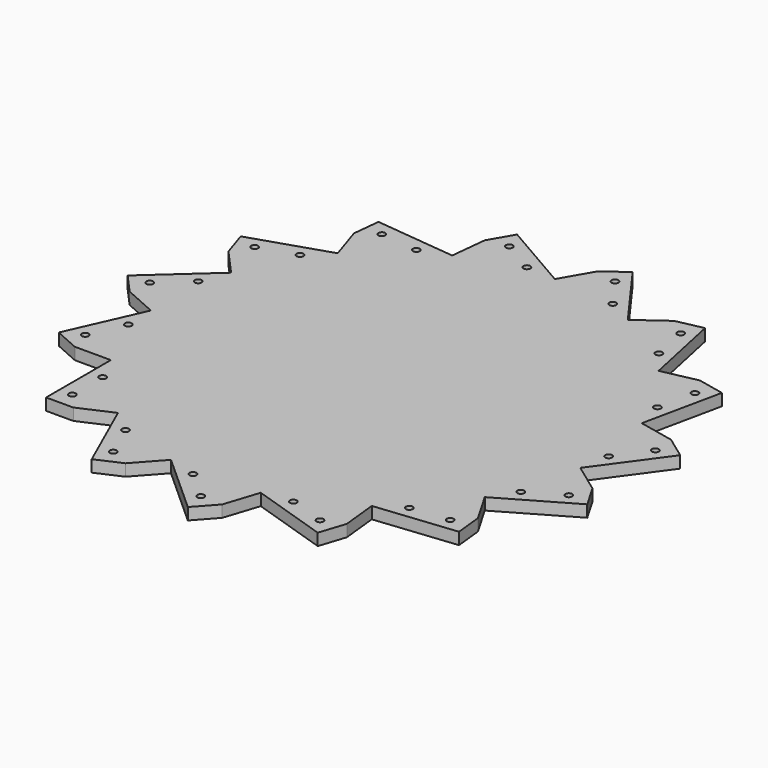
from build123d import *

# Parameters (mm, degrees)
F0_R     = 1.45
F1_DEPTH = 5


# Not quite as in the source:
# - ends of sketch curves that miss each other by under 0.0002 mm in the source are joined


with BuildPart() as f1:
    # F0 (on Top) → F1 (new body)
    with BuildSketch(Plane.XY):
        Polygon((-0.3545266845, 90.9670817697), (-29.9807621135, 108.0717967697), (-35.7307621135, 98.1125046262), (-37.3235262825, 82.9583658326), (-71.3455488748, 86.5342244993), (-72.5476262023, 75.0972227026), (-67.8389451324, 60.6053924919), (-100.3740420816, 50.0340986743), (-96.8203466463, 39.0969487369), (-86.6243940714, 27.7731962067), (-112.046951543, 4.8826226429), (-104.3519495698, -3.6635428501), (-90.4316983176, -9.8612380143), (-104.345925168, -41.1131032006), (-93.8401524051, -45.790574596), (-78.6025403784, -45.790574596), (-78.6025403784, -80), (-67.1025403784, -80), (-53.1822891262, -73.8023048358), (-39.2680622758, -105.0541700222), (-28.7622895129, -100.3766986268), (-18.5663369381, -89.0529460966), (6.8562205334, -111.9435196603), (14.5512225065, -103.3973541673), (19.2599035765, -88.9055239566), (51.7950005256, -99.4768177743), (55.3486959609, -88.5396678369), (53.7559317919, -73.3855290433), (87.7779543842, -69.8096703765), (86.5758770566, -58.3726685798), (78.9570710433, -45.1765094717), (108.583302492, -28.0717967697), (102.833302492, -18.1125046262), (90.5058154087, -9.1560609968), (110.6136111506, 18.5199455228), (101.3099157153, 25.2794759242), (86.4052820705, 28.4475536047), (93.5178215482, 61.9094209861), (82.2691241397, 64.3004054305), (67.364490495, 61.13232775), (60.2519510173, 94.5941951314), (49.0032536089, 92.203210687), (36.6757665257, 83.2467670575), (16.5679707838, 110.9227735772), (7.2642753485, 104.1632431758), align=None)
        with Locations((-73.1025403784, -73)):
            Circle(F0_R, mode=Mode.SUBTRACT)
        with Locations((-73.1025403784, -57)):
            Circle(F0_R, mode=Mode.SUBTRACT)
        with Locations((-37.0907187603, -96.4223002818)):
            Circle(F0_R, mode=Mode.SUBTRACT)
        with Locations((-6.5558921176, -92.4662191739)):
            Circle(F0_R, mode=Mode.SUBTRACT)
        with Locations((-43.5985050495, -81.8055729595)):
            Circle(F0_R, mode=Mode.SUBTRACT)
        with Locations((-96.4742686494, -36.9553365341)):
            Circle(F0_R, mode=Mode.SUBTRACT)
        with Locations((-89.9664823602, -22.3386092118)):
            Circle(F0_R, mode=Mode.SUBTRACT)
        with Locations((5.33442509, -103.1723088757)):
            Circle(F0_R, mode=Mode.SUBTRACT)
        with Locations((31.6202941199, -87.138616064)):
            Circle(F0_R, mode=Mode.SUBTRACT)
        with Locations((46.8371983806, -92.082887974)):
            Circle(F0_R, mode=Mode.SUBTRACT)
        with Locations((64.3290442427, -66.7439546071)):
            Circle(F0_R, mode=Mode.SUBTRACT)
        with Locations((80.2413945686, -65.0714991949)):
            Circle(F0_R, mode=Mode.SUBTRACT)
        with Locations((85.9147182049, -34.8086570489)):
            Circle(F0_R, mode=Mode.SUBTRACT)
        with Locations((99.7711246655, -26.8086570489)):
            Circle(F0_R, mode=Mode.SUBTRACT)
        with Locations((-103.1647194297, 5.4792403473)):
            Circle(F0_R, mode=Mode.SUBTRACT)
        with Locations((-91.274402222, 16.185330049)):
            Circle(F0_R, mode=Mode.SUBTRACT)
        with Locations((-92.0170529985, 46.9664067953)):
            Circle(F0_R, mode=Mode.SUBTRACT)
        with Locations((-76.8001487377, 51.9106787053)):
            Circle(F0_R, mode=Mode.SUBTRACT)
        with Locations((-64.9588021552, 80.3326548319)):
            Circle(F0_R, mode=Mode.SUBTRACT)
        with Locations((-49.0464518293, 78.6601994197)):
            Circle(F0_R, mode=Mode.SUBTRACT)
        with Locations((-12.8121778265, 91.8086570489)):
            Circle(F0_R, mode=Mode.SUBTRACT)
        with Locations((-26.668584287, 99.8086570489)):
            Circle(F0_R, mode=Mode.SUBTRACT)
        with Locations((92.6449568788, 3.1453735398)):
            Circle(F0_R, mode=Mode.SUBTRACT)
        with Locations((102.0495209155, 16.0896454498)):
            Circle(F0_R, mode=Mode.SUBTRACT)
        with Locations((83.3560408553, 40.5555404687)):
            Circle(F0_R, mode=Mode.SUBTRACT)
        with Locations((25.6374381175, 89.0825638189)):
            Circle(F0_R, mode=Mode.SUBTRACT)
        with Locations((16.2328740808, 102.0268357289)):
            Circle(F0_R, mode=Mode.SUBTRACT)
        with Locations((59.6541081021, 70.953286015)):
            Circle(F0_R, mode=Mode.SUBTRACT)
        with Locations((86.6826279084, 56.2059020804)):
            Circle(F0_R, mode=Mode.SUBTRACT)
        with Locations((56.327521049, 86.6036476267)):
            Circle(F0_R, mode=Mode.SUBTRACT)
    extrude(amount=F1_DEPTH)


solid = f1.part
